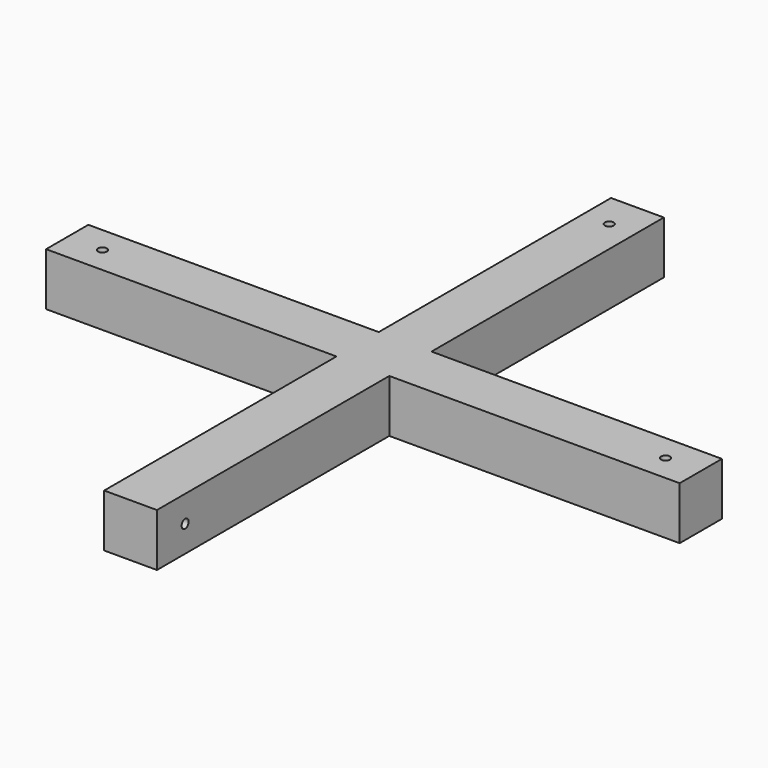
from build123d import *

# Parameters (mm, degrees)
F0_W     = 9.525
F0_H     = 52.3875
F0_W_2   = 52.3875
F0_H_2   = 9.525
F1_DEPTH = 9.525
F2_R     = 0.79375
F3_DEPTH = 9.525
F4_R     = 0.79375
F5_DEPTH = 9.525
F6_W     = 64.4
F6_H     = 21
F7_DEPTH = 11.15


# Not quite as in the source:
# - a length typed as a fraction of an inch, garbled in the dataset ("3 / 203.2 mm" for 3/8 in), is restored


with BuildPart() as f1:
    # F0 (on Top) → F1 (new body)
    with BuildSketch(Plane.XY):
        with Locations((0, 30.95625)):
            Rectangle(F0_W, F0_H)
        with Locations((30.95625, 0)):
            Rectangle(F0_W_2, F0_H_2)
        Rectangle(F0_W, F0_H_2)
        with Locations((0, -30.95625)):
            Rectangle(F0_W, F0_H)
        with Locations((-30.95625, 0)):
            Rectangle(F0_W_2, F0_H_2)
    extrude(amount=F1_DEPTH)

    # F2 (on face) → F3 (cut)
    with BuildSketch(Plane.XY.offset(9.525)):
        with Locations((0, 50.8)):
            Circle(F2_R)
        with Locations((50.8, 0)):
            Circle(F2_R)
        with Locations((-50.8, 0)):
            Circle(F2_R)
    extrude(amount=-F3_DEPTH, mode=Mode.SUBTRACT)

    # F4 (on face) → F5 (cut)
    with BuildSketch(Plane(origin=(-4.7625, 0, 0), x_dir=(0, -1, 0), z_dir=(-1, 0, 0))):
        with Locations((50.8, 4.7625)):
            Circle(F4_R)
    extrude(amount=-F5_DEPTH, mode=Mode.SUBTRACT)


with BuildPart() as f7:
    # F6 (on Top) → F7 (new body, symmetric)
    with BuildSketch(Plane.XY):
        with Locations((0, 0.8)):
            Rectangle(F6_W, F6_H)
    extrude(amount=F7_DEPTH, both=True)


solid = f1.part
